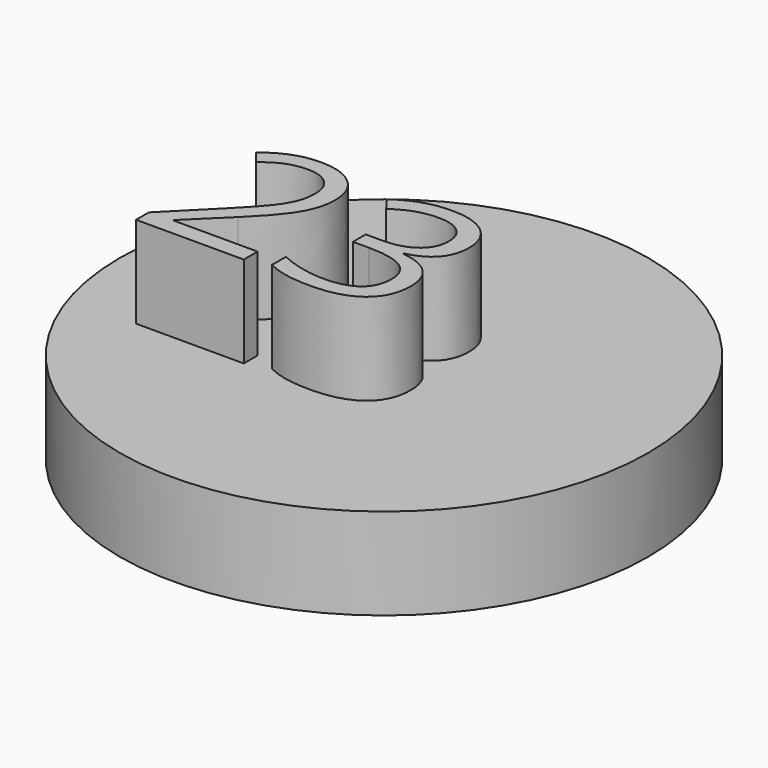
from build123d import *

# Parameters (mm, degrees)
F0_R         = 73.3348771631
F1_DEPTH     = 25.4
F2_TEXT_SIZE = 63.7262800915
F3_DEPTH     = 25.4


# Not quite as in the source:
# - Text() gives the source's letters only with a copy of the font that has no kerning and outlines rounded to 1/6400 em; it was checked with that copy


with BuildPart() as f1:
    # F0 (on Top) → F1 (new body)
    with BuildSketch(Plane.XY):
        with Locations((2.2895033471, 0)):
            Circle(F0_R)
    extrude(amount=F1_DEPTH)

    # F2 (on face) → F3 (join)
    with BuildSketch(Plane.XY.offset(25.4)):
        with Locations((-52.1140806377, -21.9401996583)):
            Text('23', F2_TEXT_SIZE, font='Open Sans', text_align=(TextAlign.LEFT, TextAlign.BOTTOM))
    extrude(amount=F3_DEPTH)


solid = f1.part
